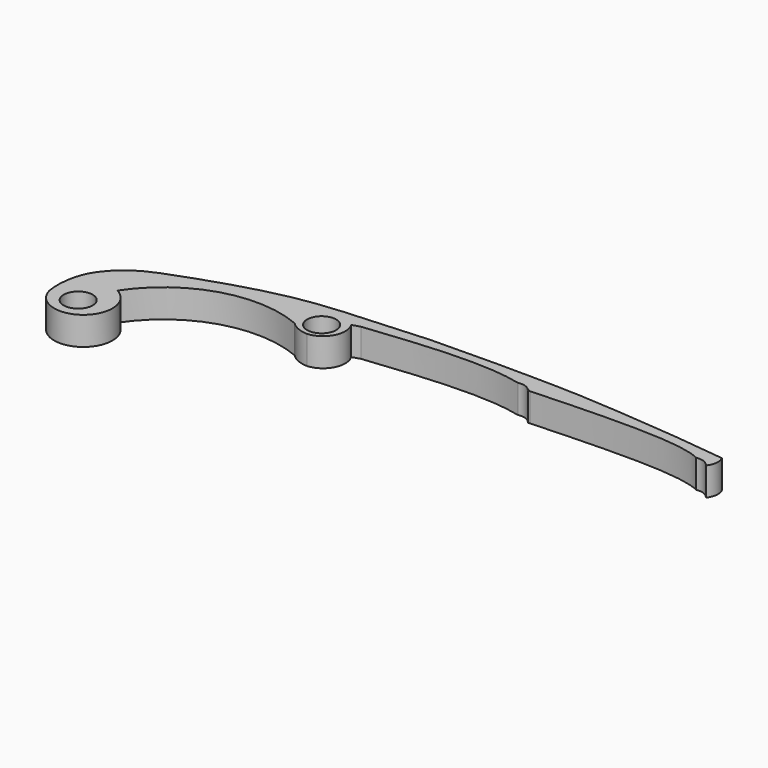
from build123d import *

# Parameters (mm, degrees)
F0_R     = 2.1
F1_DEPTH = 4.1


# Not quite as in the source:
# - the dataset's text gives a spline's control points without its knots; the knots are read off the source's solid


with BuildPart() as f1:
    # F0 (on Top) → F1 (new body)
    with BuildSketch(Plane.XY):
        with BuildLine():
            add(Edge.make_bspline(
                [(-7.1889940943, 11.3371111296), (-4.0400674757, 11.378726928), (-0.8911408571, 11.4203427264), (2.2577857615, 11.4619585248)],
                knots=[0.0025744578, 0.0025744578, 0.0025744578, 0.0025744578, 0.9981985586, 0.9981985586, 0.9981985586, 0.9981985586], degree=3))
            add(Edge.make_bspline(
                [(-7.1889940943, 11.3371111296), (-8.7243380234, 11.2416990231), (-11.0311154467, 11.0983567929), (-14.0552941607, 10.9070068206), (-17.0364840295, 10.7152017294), (-19.8957827411, 10.5227751645), (-22.6755680541, 10.2254472092), (-24.7351040641, 9.9221224701), (-26.7907840734, 9.5226800469), (-28.7930725745, 9.0595604731), (-30.7009918926, 8.5581161043), (-32.4611472882, 8.0493632371), (-34.0928691245, 7.5399082887), (-35.6448312044, 7.0260920816), (-37.1607478855, 6.5079303839), (-38.6478053455, 5.9835690127), (-39.8743681253, 5.5332793467), (-40.8467259962, 5.1646139076), (-41.7960653414, 4.7845249787), (-42.9412331822, 4.2634047579), (-44.2283369213, 3.5006412719), (-45.4526195393, 2.5238601501), (-46.3467921373, 1.5924900737), (-46.9440085195, 0.8150763514), (-47.4224819266, 0.0716833781), (-47.6925333314, -0.4904090932), (-47.8380102388, -0.8639908212)],
                knots=[0.0001645527, 0.0001645527, 0.0001645527, 0.0001645527, 0.03125, 0.046875, 0.0625, 0.09375, 0.109375, 0.125, 0.140625, 0.15625, 0.171875, 0.1875, 0.203125, 0.21875, 0.234375, 0.25, 0.265625, 0.2734375, 0.28125, 0.296875, 0.3125, 0.328125, 0.34375, 0.3515625, 0.359375, 0.373459546, 0.373459546, 0.373459546, 0.373459546], degree=3))
            add(Edge.make_bspline(
                [(-47.8380102388, -0.8639908212), (-47.8539213294, -0.9048501769), (-48.0274581717, -1.3617547655), (-48.2807207722, -2.2706204398), (-48.4770009887, -3.7150176775), (-48.4798207479, -4.9756086404), (-48.3888275454, -5.7962324568), (-48.3392794649, -6.1066755823), (-48.3299230612, -6.1621975504)],
                knots=[0.373459546, 0.373459546, 0.373459546, 0.373459546, 0.375, 0.390625, 0.40625, 0.421875, 0.4296875, 0.4313894643, 0.4313894643, 0.4313894643, 0.4313894643], degree=3))
            ThreePointArc((-48.3299230612, -6.1621975504), (-41.6093586104, -8.374837019), (-42.3299329619, -1.3361913709))
            ThreePointArc((-42.3299329619, -1.3361913709), (-33.1444175869, 5.5275459689), (-21.6926677793, 4.9427303382))
            ThreePointArc((-21.6926677793, 4.9427303382), (-20.4406705014, 4.0833356397), (-18.9537504594, 3.7749118723))
            ThreePointArc((-18.9537504594, 3.7749118723), (-16.3562817519, 5.4925025893), (-16.4336573959, 8.6055356067))
            add(Edge.make_bspline(
                [(-15.3179860369, 8.9560919431), (-15.6898764899, 8.839239831), (-16.0617669429, 8.7223877188), (-16.4336573959, 8.6055356067)],
                knots=[0, 0, 0, 0, 1.1694495826, 1.1694495826, 1.1694495826, 1.1694495826], degree=3))
            add(Edge.make_bspline(
                [(-15.3179860369, 8.9560919431), (-7.0361622279, 9.8603205112), (1.2450933884, 10.7540884183), (7.1086706108, 9.3142706211)],
                knots=[0, 0, 0, 0, 0.5814306684, 0.5814306684, 0.5814306684, 0.5814306684], degree=3))
            ThreePointArc((7.1086706108, 9.3142706211), (8.1397564178, 9.2807598726), (9.0169736045, 8.7378501942))
            add(Edge.make_bspline(
                [(9.0169736045, 8.7378501942), (9.1112334208, 8.7038678093), (9.2048591167, 8.6692727004), (9.2978690964, 8.6340825262)],
                knots=[0.6474492811, 0.6474492811, 0.6474492811, 0.6474492811, 0.6576832175, 0.6576832175, 0.6576832175, 0.6576832175], degree=3))
            add(Edge.make_bspline(
                [(9.2978690964, 8.6340825262), (9.3620169205, 8.6098123015), (9.4258718675, 8.5852590228), (9.4894399752, 8.5604284832)],
                knots=[0.6576832175, 0.6576832175, 0.6576832175, 0.6576832175, 0.664741436, 0.664741436, 0.664741436, 0.664741436], degree=3))
            add(Edge.make_bspline(
                [(9.4894399752, 8.5604284832), (20.1786312058, 9.0171598272), (30.7897103436, 9.4434976677), (34.3049085784, 7.5800661268)],
                knots=[0.0078728095, 0.0078728095, 0.0078728095, 0.0078728095, 0.7340214047, 0.7340214047, 0.7340214047, 0.7340214047], degree=3))
            ThreePointArc((34.3049085784, 7.5800661268), (35.4462954706, 7.4859898214), (36.3489343996, 6.7811087302))
            ThreePointArc((36.3489343996, 6.7811087302), (36.8790497693, 8.0037841101), (36.6502768797, 9.3166513367))
            add(Edge.make_bspline(
                [(36.6502768797, 9.3166513367), (35.8646692204, 9.4102452527), (34.5771705441, 9.5641656546), (32.8453284038, 9.766858119), (31.4810593515, 9.9216959685), (30.2216638222, 10.0570259134), (29.0749710159, 10.1710606279), (27.998427122, 10.2705354697), (26.9593851329, 10.3605177789), (25.9224275902, 10.4465645091), (24.8546312229, 10.5337851633), (23.7183846338, 10.6284306145), (22.0947419096, 10.7659145801), (19.8690501247, 10.947846215), (17.3823459067, 11.1199052699), (15.2379483396, 11.23710443), (13.5543144395, 11.3113741003), (11.7890118212, 11.36769996), (9.9748087559, 11.4062922205), (8.1910240467, 11.4310364541), (6.5067223519, 11.4450690607), (4.9932998476, 11.4517588504), (3.72086677, 11.4544341193), (2.9197217826, 11.456089603), (2.4761636021, 11.4587356227), (2.3200545408, 11.4607049569), (2.2577857615, 11.4619585248)],
                knots=[0.6753696694, 0.6753696694, 0.6753696694, 0.6753696694, 0.6857638921, 0.692086291, 0.6984086899, 0.7047310889, 0.7110534878, 0.7173758867, 0.7236982857, 0.7300206846, 0.7363430835, 0.7426654824, 0.7489878814, 0.7616326792, 0.7742774771, 0.780599876, 0.7869222749, 0.7932446739, 0.7995670728, 0.8058894717, 0.8122118707, 0.8185342696, 0.8248566685, 0.8311790674, 0.8343402669, 0.8372170533, 0.8372170533, 0.8372170533, 0.8372170533], degree=3))
        make_face()
        with Locations((-44.3371695162, -5.9176166552)):
            Circle(F0_R, mode=Mode.SUBTRACT)
        with Locations((-19.0713156642, 6.5468703386)):
            Circle(F0_R, mode=Mode.SUBTRACT)
        with BuildLine():
            add(Edge.make_bspline(
                [(9.1756523659, 8.5470149257), (9.2802513314, 8.5514876104), (9.3848493925, 8.5559595017), (9.4894399752, 8.5604284832)],
                knots=[0.0007676597, 0.0007676597, 0.0007676597, 0.0007676597, 0.0078728095, 0.0078728095, 0.0078728095, 0.0078728095], degree=3))
            add(Edge.make_bspline(
                [(9.2978690964, 8.6340825262), (9.3620169205, 8.6098123015), (9.4258718675, 8.5852590228), (9.4894399752, 8.5604284832)],
                knots=[0.6576832175, 0.6576832175, 0.6576832175, 0.6576832175, 0.664741436, 0.664741436, 0.664741436, 0.664741436], degree=3))
            ThreePointArc((9.2978690964, 8.6340825262), (9.2334907266, 8.5946425284), (9.1672526158, 8.5584126983))
            ThreePointArc((9.1672526158, 8.5584126983), (9.1714625769, 8.5527212451), (9.1756523659, 8.5470149257))
        make_face()
    extrude(amount=F1_DEPTH)


solid = f1.part
